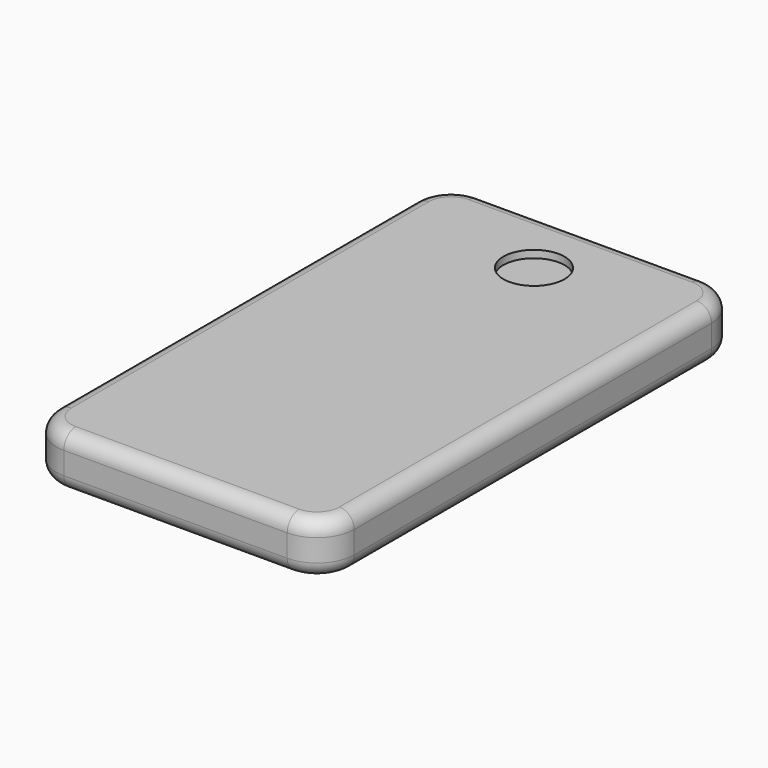
from build123d import *

# Parameters (mm, degrees)
F0_W         = 40
F0_H         = 70
F1_DEPTH     = 7
F2_R         = 5
F3_R         = 2
F4_DEPTH     = 5
F5_T1_DEPTH  = 30
F5_T3_DEPTH  = 60
F5_T6_ANGLE  = 90
F5_T8_ANGLE  = 90
F5_T10_ANGLE = 90
F5_T12_ANGLE = 90
F5_T14_ANGLE = 90
F5_T16_ANGLE = 90
F5_T18_ANGLE = 90
F5_T20_ANGLE = 90
F6_R         = 4.1045895756
F7_DEPTH     = 1
F8_R         = 0.5
F9_DEPTH     = 5
F11_DEPTH    = 5
F12_R        = 0.5
F13_DEPTH    = 5


# Not quite as in the source:
# - a fillet or chamfer that OpenCascade refuses, or shapes differently, is made with other operations: its cross-section is extruded or revolved along the edge and cut away or added


with BuildPart() as f1:
    # F0 (on Top) → F1 (new body)
    with BuildSketch(Plane.XY):
        with Locations((20, 35)):
            Rectangle(F0_W, F0_H)
    extrude(amount=F1_DEPTH)

    # F2
    f2_edges = [f1.edges().sort_by_distance(p)[0] for p in [
        (40, 0, 3.5),
        (0, 0, 3.5),
        (40, 70, 3.5),
        (0, 70, 3.5),
    ]]
    fillet(f2_edges, radius=F2_R)

    # F3 (on face) → F4 (cut)
    with BuildSketch(Plane(origin=(0, 70, 0), x_dir=(-1, 0, 0), z_dir=(0, 1, 0))):
        with Locations((-31, 3.5)):
            Circle(F3_R)
    extrude(amount=-F4_DEPTH, mode=Mode.SUBTRACT)

    # F5: fillet of radius 2 on 16 edges, made by hand

    # F5_s2 → F5_t1 (cut)
    with BuildSketch(Plane.YZ.offset(5)):
        with BuildLine():
            ThreePointArc((68, 7), (69.4142135624, 6.4142135624), (70, 5))
            Line((70, 5), (70, 7))
            Line((70, 7), (68, 7))
        make_face()
        with BuildLine():
            ThreePointArc((68, 0), (69.4142135624, 0.5857864376), (70, 2))
            Line((70, 2), (70, 0))
            Line((70, 0), (68, 0))
        make_face()
        with BuildLine():
            ThreePointArc((2, 0), (0.5857864376, 0.5857864376), (0, 2))
            Line((0, 2), (0, 0))
            Line((0, 0), (2, 0))
        make_face()
        with BuildLine():
            ThreePointArc((2, 7), (0.5857864376, 6.4142135624), (0, 5))
            Line((0, 5), (0, 7))
            Line((0, 7), (2, 7))
        make_face()
    extrude(amount=F5_T1_DEPTH, mode=Mode.SUBTRACT)

    # F5_s4 → F5_t3 (cut)
    with BuildSketch(Plane.XZ.offset(-65)):
        with BuildLine():
            ThreePointArc((0, 2), (0.5857864376, 0.5857864376), (2, 0))
            Line((2, 0), (0, 0))
            Line((0, 0), (0, 2))
        make_face()
        with BuildLine():
            ThreePointArc((0, 5), (0.5857864376, 6.4142135624), (2, 7))
            Line((2, 7), (0, 7))
            Line((0, 7), (0, 5))
        make_face()
        with BuildLine():
            ThreePointArc((38, 0), (39.4142135624, 0.5857864376), (40, 2))
            Line((40, 2), (40, 0))
            Line((40, 0), (38, 0))
        make_face()
        with BuildLine():
            ThreePointArc((38, 7), (39.4142135624, 6.4142135624), (40, 5))
            Line((40, 5), (40, 7))
            Line((40, 7), (38, 7))
        make_face()
    extrude(amount=F5_T3_DEPTH, mode=Mode.SUBTRACT)

    # F5_s5 → F5_t6 (revolve, cut)
    with BuildSketch(Plane.XZ.offset(-65)):
        with BuildLine():
            ThreePointArc((2, 0), (0.5857864376, 0.5857864376), (0, 2))
            Line((0, 2), (0, 0))
            Line((0, 0), (2, 0))
        make_face()
    revolve(axis=Axis((5, 65, 0), (0, 0, -1)), revolution_arc=F5_T6_ANGLE, mode=Mode.SUBTRACT)

    # F5_s7 → F5_t8 (revolve, cut)
    with BuildSketch(Plane.XZ.offset(-5)):
        with BuildLine():
            ThreePointArc((2, 0), (0.5857864376, 0.5857864376), (0, 2))
            Line((0, 2), (0, 0))
            Line((0, 0), (2, 0))
        make_face()
    revolve(axis=Axis((5, 5, 0), (0, 0, 1)), revolution_arc=F5_T8_ANGLE, mode=Mode.SUBTRACT)

    # F5_s9 → F5_t10 (revolve, cut)
    with BuildSketch(Plane.XZ.offset(-65)):
        with BuildLine():
            ThreePointArc((38, 0), (39.4142135624, 0.5857864376), (40, 2))
            Line((40, 2), (40, 0))
            Line((40, 0), (38, 0))
        make_face()
    revolve(axis=Axis((35, 65, 0), (0, 0, 1)), revolution_arc=F5_T10_ANGLE, mode=Mode.SUBTRACT)

    # F5_s11 → F5_t12 (revolve, cut)
    with BuildSketch(Plane.YZ.offset(35)):
        with BuildLine():
            ThreePointArc((2, 0), (0.5857864376, 0.5857864376), (0, 2))
            Line((0, 2), (0, 0))
            Line((0, 0), (2, 0))
        make_face()
    revolve(axis=Axis((35, 5, 0), (0, 0, 1)), revolution_arc=F5_T12_ANGLE, mode=Mode.SUBTRACT)

    # F5_s13 → F5_t14 (revolve, cut)
    with BuildSketch(Plane.XZ.offset(-65)):
        with BuildLine():
            ThreePointArc((0, 5), (0.5857864376, 6.4142135624), (2, 7))
            Line((2, 7), (0, 7))
            Line((0, 7), (0, 5))
        make_face()
    revolve(axis=Axis((5, 65, 7), (0, 0, -1)), revolution_arc=F5_T14_ANGLE, mode=Mode.SUBTRACT)

    # F5_s15 → F5_t16 (revolve, cut)
    with BuildSketch(Plane.XZ.offset(-5)):
        with BuildLine():
            ThreePointArc((0, 5), (0.5857864376, 6.4142135624), (2, 7))
            Line((2, 7), (0, 7))
            Line((0, 7), (0, 5))
        make_face()
    revolve(axis=Axis((5, 5, 7), (0, 0, 1)), revolution_arc=F5_T16_ANGLE, mode=Mode.SUBTRACT)

    # F5_s17 → F5_t18 (revolve, cut)
    with BuildSketch(Plane.XZ.offset(-65)):
        with BuildLine():
            ThreePointArc((38, 7), (39.4142135624, 6.4142135624), (40, 5))
            Line((40, 5), (40, 7))
            Line((40, 7), (38, 7))
        make_face()
    revolve(axis=Axis((35, 65, 7), (0, 0, 1)), revolution_arc=F5_T18_ANGLE, mode=Mode.SUBTRACT)

    # F5_s19 → F5_t20 (revolve, cut)
    with BuildSketch(Plane.YZ.offset(35)):
        with BuildLine():
            ThreePointArc((2, 7), (0.5857864376, 6.4142135624), (0, 5))
            Line((0, 5), (0, 7))
            Line((0, 7), (2, 7))
        make_face()
    revolve(axis=Axis((35, 5, 7), (0, 0, 1)), revolution_arc=F5_T20_ANGLE, mode=Mode.SUBTRACT)

    # F6 (on face) → F7 (cut)
    with BuildSketch(Plane.XY.offset(7)):
        with Locations((20, 60.1752847433)):
            Circle(F6_R)
    extrude(amount=-F7_DEPTH, mode=Mode.SUBTRACT)

    # F8 (on face) → F9 (cut)
    with BuildSketch(Plane(origin=(0, 70, 0), x_dir=(-1, 0, 0), z_dir=(0, 1, 0))):
        with Locations((-28, 3.5)):
            Circle(F8_R)
    extrude(amount=-F9_DEPTH, mode=Mode.SUBTRACT)

    # F10 (on face) → F11 (cut)
    with BuildSketch(Plane(origin=(0, 70, 0), x_dir=(-1, 0, 0), z_dir=(0, 1, 0))):
        with BuildLine():
            Line((-17.383011058, 4.4047813863), (-22.5439444184, 4.4047813863))
            ThreePointArc((-22.5439444184, 4.4047813863), (-23.4822960338, 3.4664297709), (-22.5439444184, 2.5280781556))
            Line((-22.5439444184, 2.5280781556), (-17.383011058, 2.5280781556))
            ThreePointArc((-17.383011058, 2.5280781556), (-16.4446594426, 3.4664297709), (-17.383011058, 4.4047813863))
        make_face()
    extrude(amount=-F11_DEPTH, mode=Mode.SUBTRACT)

    # F12 (on face) → F13 (cut)
    with BuildSketch(Plane(origin=(0, 70, 0), x_dir=(-1, 0, 0), z_dir=(0, 1, 0))):
        with Locations((-6.5, 3.5)):
            Circle(F12_R)
        with Locations((-8, 3.5)):
            Circle(F12_R)
        with Locations((-9.5, 3.5)):
            Circle(F12_R)
        with Locations((-11, 3.5)):
            Circle(F12_R)
    extrude(amount=-F13_DEPTH, mode=Mode.SUBTRACT)


solid = f1.part
